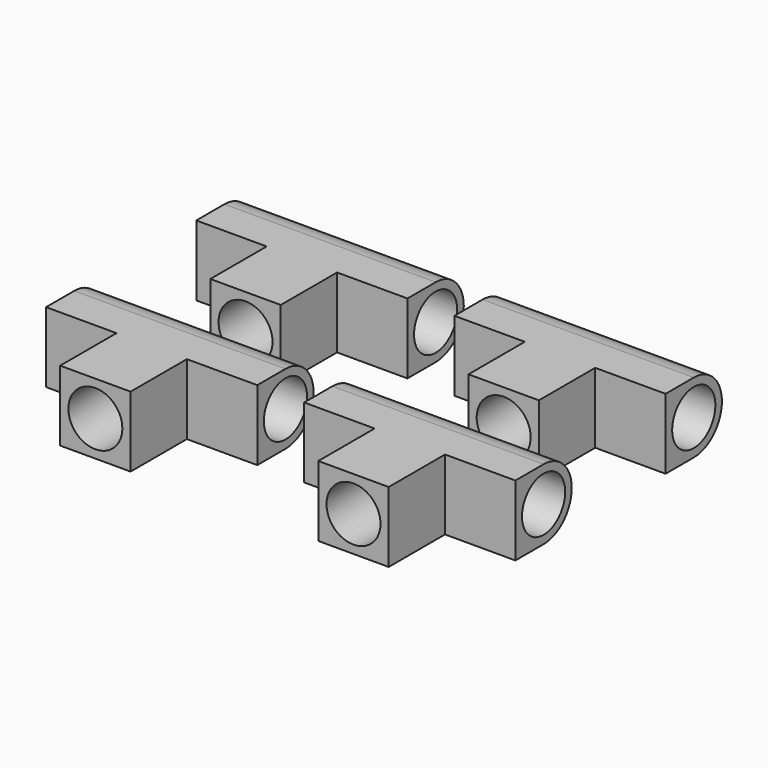
from build123d import *

# Parameters (mm, degrees)
F1_DEPTH = 30
F3_R     = 11.5
F4_DEPTH = 30
F2_R     = 11.5
F5_DEPTH = 90
F6_R     = 14.99999


# Not quite as in the source:
# - a fillet or chamfer is up to 0.001 mm smaller than in the source, because OpenCascade refuses the exact size


with BuildPart() as f1:
    # F0 (on Top) → F1 (new body)
    with BuildSketch(Plane.XY):
        Polygon((15, -15), (45, -15), (45, 15), (-45, 15), (-45, -15), (-15, -15), align=None)
        Polygon((15, -45), (15, -15), (-15, -15), (-15, -45), (0, -45), align=None)
    extrude(amount=F1_DEPTH)

    # F3 (on face) → F4 (cut)
    with BuildSketch(Plane.XZ.offset(45)):
        with Locations((0, 15)):
            Circle(F3_R)
    extrude(amount=-F4_DEPTH, mode=Mode.SUBTRACT)

    # F2 (on face) → F5 (cut)
    with BuildSketch(Plane(origin=(-45, 0, 0), x_dir=(0, -1, 0), z_dir=(-1, 0, 0))):
        with Locations((0, 15)):
            Circle(F2_R)
    extrude(amount=-F5_DEPTH, mode=Mode.SUBTRACT)

    # F6 (radius 15 in the source; OpenCascade refuses exactly that, so slightly less here)
    f6_edges = [f1.edges().sort_by_distance(p)[0] for p in [
        (0, 15, 0),
        (0, 15, 30),
    ]]
    fillet(f6_edges, radius=F6_R)


with BuildPart() as f7_1:
    # F7: copy of F1
    add(f1.part.moved(Location((0, 80, 0))))


with BuildPart() as f8_1:
    # F8: copy of F1
    add(f1.part.moved(Location((110, 80, 0))))


with BuildPart() as f9_1:
    # F9: copy of F1
    add(f1.part.moved(Location((110, 0, 0))))


solid = Compound([f1.part, f7_1.part, f8_1.part, f9_1.part])
